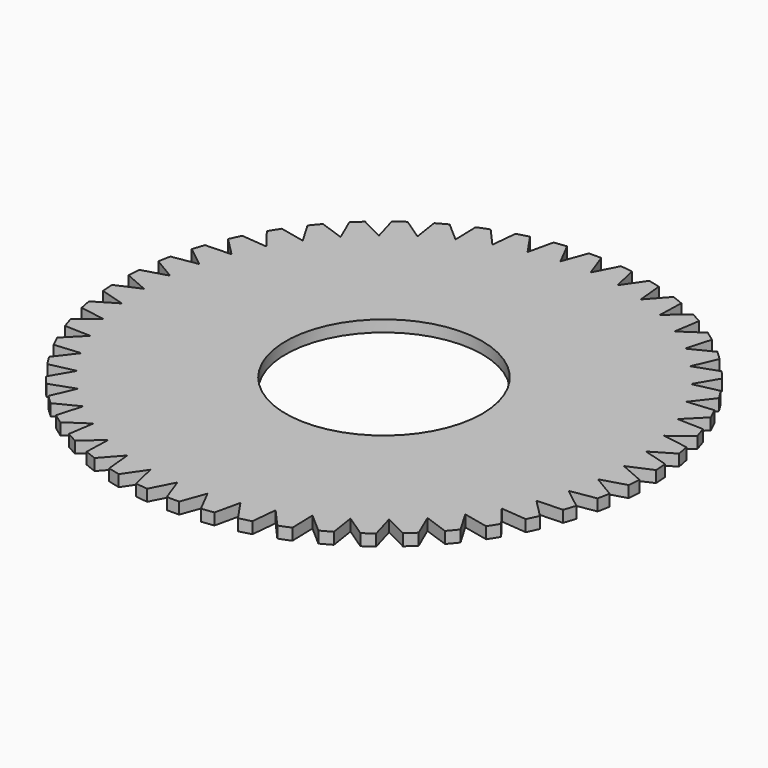
from build123d import *

# Parameters (mm, degrees)
F0_R     = 17.4625
F0_R_2   = 6.5024
F1_DEPTH = 0.762
F3_DEPTH = 0.762


with BuildPart() as f1:
    # F0 (on Top) → F1 (new body)
    with BuildSketch(Plane.XY):
        Circle(F0_R)
        Circle(F0_R_2, mode=Mode.SUBTRACT)
    extrude(amount=F1_DEPTH)

    # F2 (on face) → F3 (cut, through all)
    with BuildSketch(Plane.XY.offset(0.762)):
        with BuildLine():
            Line((17.44898324, 0.6869426038), (15.875, 0))
            Line((15.875, 0), (17.44898324, -0.6869426038))
            ThreePointArc((17.44898324, -0.6869426038), (17.459120483, -0.3435377868), (17.4625, 0))
            ThreePointArc((17.4625, 0), (17.459120483, 0.3435377868), (17.44898324, 0.6869426038))
        make_face()
        with BuildLine():
            Line((17.2252960576, 2.8684633481), (15.7498208834, 1.9896650828))
            Line((15.7498208834, 1.9896650828), (17.3974895332, 1.5054116357))
            ThreePointArc((17.3974895332, 1.5054116357), (17.3645068048, 1.8473791366), (17.3248029717, 2.1886315911))
            ThreePointArc((17.3248029717, 2.1886315911), (17.2783934015, 2.529036914), (17.2252960576, 2.8684633481))
        make_face()
        with BuildLine():
            Line((16.7299556664, 5.0047467118), (15.3762576829, 3.9479519587))
            Line((15.3762576829, 3.9479519587), (17.0716270237, 3.6740246344))
            ThreePointArc((17.0716270237, 3.6740246344), (16.9960444814, 4.0091617875), (16.9138834512, 4.3427471546))
            ThreePointArc((16.9138834512, 4.3427471546), (16.8251757345, 4.6746516184), (16.7299556664, 5.0047467118))
        make_face()
        with BuildLine():
            Line((15.9707738805, 7.0621022302), (14.7602017135, 5.8439772739))
            Line((14.7602017135, 5.8439772739), (16.4765347579, 5.7846960699))
            ThreePointArc((16.4765347579, 5.7846960699), (16.3595443834, 6.1077175619), (16.2362218848, 6.4283750013))
            ThreePointArc((16.2362218848, 6.4283750013), (16.1066149953, 6.7465442742), (15.9707738805, 7.0621022302))
        make_face()
        with BuildLine():
            Line((14.9597234499, 9.0080841777), (13.9113685457, 7.6478395764))
            Line((13.9113685457, 7.6478395764), (15.6215976964, 7.8041393927))
            ThreePointArc((15.6215976964, 7.8041393927), (15.4650444979, 8.1099509819), (15.3025054003, 8.412623534))
            ThreePointArc((15.3025054003, 8.412623534), (15.134043316, 8.7120398966), (14.9597234499, 9.0080841777))
        make_face()
        with BuildLine():
            Line((13.712749244, 10.8120032566), (12.8431447857, 9.3310908801))
            Line((12.8431447857, 9.3310908801), (14.5202987074, 9.7005067753))
            ThreePointArc((14.5202987074, 9.7005067753), (14.3266516222, 9.9842856302), (14.1274592643, 10.2641999682))
            ThreePointArc((14.1274592643, 10.2641999682), (13.9227987329, 10.5401414456), (13.712749244, 10.8120032566))
        make_face()
        with BuildLine():
            Line((12.249516791, 12.4454105853), (11.5723769603, 10.8671853066))
            Line((11.5723769603, 10.8671853066), (13.1900059337, 11.4438913713))
            ThreePointArc((13.1900059337, 11.4438913713), (12.9623188922, 11.7011621298), (12.7296146563, 11.9539038373))
            ThreePointArc((12.7296146563, 11.9539038373), (12.4919832968, 12.2020186676), (12.249516791, 12.4454105853))
        make_face()
        with BuildLine():
            Line((10.5931021406, 13.8825463546), (10.1191058373, 12.2318977291))
            Line((10.1191058373, 12.2318977291), (11.6516988871, 13.0067989641))
            ThreePointArc((11.6516988871, 13.0067989641), (11.3935626498, 13.2335043127), (11.131016421, 13.455087502))
            ThreePointArc((11.131016421, 13.455087502), (10.8641618217, 13.671462766), (10.5931021406, 13.8825463546))
        make_face()
        with BuildLine():
            Line((8.7696279415, 15.1007460749), (8.5062503703, 13.4037058173))
            Line((8.5062503703, 13.4037058173), (9.9296375887, 14.3645815674))
            ThreePointArc((9.9296375887, 14.3645815674), (9.6451231184, 14.5571462273), (9.3568754073, 14.7440763991))
            ThreePointArc((9.3568754073, 14.7440763991), (9.0650060247, 14.9252997297), (8.7696279415, 15.1007460749))
        make_face()
        with BuildLine():
            Line((6.807851471, 16.0807980087), (6.7592462536, 14.3641294579))
            Line((6.7592462536, 14.3641294579), (8.0509799739, 15.4958261384))
            ThreePointArc((8.0509799739, 15.4958261384), (7.7445742336, 15.6512132498), (7.435170879, 15.8005424037))
            ThreePointArc((7.435170879, 15.8005424037), (7.1228896676, 15.9437558007), (6.807851471, 16.0807980087))
        make_face()
        with BuildLine():
            Line((4.7387111161, 16.8072461518), (4.9056447857, 15.0980221962))
            Line((4.9056447857, 15.0980221962), (6.0453535954, 16.3826922744))
            ThreePointArc((6.0453535954, 16.3826922744), (5.7218887868, 16.4984512898), (5.3962092643, 16.6078244158))
            ThreePointArc((5.3962092643, 16.6078244158), (5.0684410854, 16.7107693184), (4.7387111161, 16.8072461518))
        make_face()
        with BuildLine():
            Line((2.594838456, 17.268633983), (2.974678369, 15.5938101053))
            Line((2.974678369, 15.5938101053), (3.9443883794, 17.0111935667))
            ThreePointArc((3.9443883794, 17.0111935667), (3.6089657357, 17.0854988973), (3.272146206, 17.1531911158))
            ThreePointArc((3.272146206, 17.1531911158), (2.9340601595, 17.2142440215), (2.594838456, 17.268633983))
        make_face()
        with BuildLine():
            Line((0.4100436434, 17.4576851404), (0.9967994975, 15.8436743138))
            Line((0.9967994975, 15.8436743138), (1.7812178024, 17.3714181744))
            ThreePointArc((1.7812178024, 17.3714181744), (1.4391271391, 17.4030979808), (1.0964794473, 17.4280417452))
            ThreePointArc((1.0964794473, 17.4280417452), (0.7534073522, 17.446239813), (0.4100436434, 17.4576851404))
        make_face()
        with BuildLine():
            Line((-1.7812178024, 17.3714181744), (-0.9967994975, 15.8436743138))
            Line((-0.9967994975, 15.8436743138), (-0.4100436434, 17.4576851404))
            ThreePointArc((-0.4100436434, 17.4576851404), (-0.7534073522, 17.446239813), (-1.0964794473, 17.4280417452))
            ThreePointArc((-1.0964794473, 17.4280417452), (-1.4391271391, 17.4030979808), (-1.7812178024, 17.3714181744))
        make_face()
        with BuildLine():
            Line((-3.9443883794, 17.0111935667), (-2.974678369, 15.5938101053))
            Line((-2.974678369, 15.5938101053), (-2.594838456, 17.268633983))
            ThreePointArc((-2.594838456, 17.268633983), (-2.9340601595, 17.2142440215), (-3.272146206, 17.1531911158))
            ThreePointArc((-3.272146206, 17.1531911158), (-3.6089657357, 17.0854988973), (-3.9443883794, 17.0111935667))
        make_face()
        with BuildLine():
            Line((-6.0453535954, 16.3826922744), (-4.9056447857, 15.0980221962))
            Line((-4.9056447857, 15.0980221962), (-4.7387111161, 16.8072461518))
            ThreePointArc((-4.7387111161, 16.8072461518), (-5.0684410854, 16.7107693184), (-5.3962092643, 16.6078244158))
            ThreePointArc((-5.3962092643, 16.6078244158), (-5.7218887868, 16.4984512898), (-6.0453535954, 16.3826922744))
        make_face()
        with BuildLine():
            Line((-8.0509799739, 15.4958261384), (-6.7592462536, 14.3641294579))
            Line((-6.7592462536, 14.3641294579), (-6.807851471, 16.0807980087))
            ThreePointArc((-6.807851471, 16.0807980087), (-7.1228896676, 15.9437558007), (-7.435170879, 15.8005424037))
            ThreePointArc((-7.435170879, 15.8005424037), (-7.7445742336, 15.6512132498), (-8.0509799739, 15.4958261384))
        make_face()
        with BuildLine():
            Line((-9.9296375887, 14.3645815674), (-8.5062503703, 13.4037058173))
            Line((-8.5062503703, 13.4037058173), (-8.7696279415, 15.1007460749))
            ThreePointArc((-8.7696279415, 15.1007460749), (-9.0650060247, 14.9252997297), (-9.3568754073, 14.7440763991))
            ThreePointArc((-9.3568754073, 14.7440763991), (-9.6451231184, 14.5571462273), (-9.9296375887, 14.3645815674))
        make_face()
        with BuildLine():
            Line((-11.6516988871, 13.0067989641), (-10.1191058373, 12.2318977291))
            Line((-10.1191058373, 12.2318977291), (-10.5931021406, 13.8825463546))
            ThreePointArc((-10.5931021406, 13.8825463546), (-10.8641618217, 13.671462766), (-11.131016421, 13.455087502))
            ThreePointArc((-11.131016421, 13.455087502), (-11.3935626498, 13.2335043127), (-11.6516988871, 13.0067989641))
        make_face()
        with BuildLine():
            Line((-13.1900059337, 11.4438913713), (-11.5723769603, 10.8671853066))
            Line((-11.5723769603, 10.8671853066), (-12.249516791, 12.4454105853))
            ThreePointArc((-12.249516791, 12.4454105853), (-12.4919832968, 12.2020186676), (-12.7296146563, 11.9539038373))
            ThreePointArc((-12.7296146563, 11.9539038373), (-12.9623188922, 11.7011621298), (-13.1900059337, 11.4438913713))
        make_face()
        with BuildLine():
            Line((-14.5202987074, 9.7005067753), (-12.8431447857, 9.3310908801))
            Line((-12.8431447857, 9.3310908801), (-13.712749244, 10.8120032566))
            ThreePointArc((-13.712749244, 10.8120032566), (-13.9227987329, 10.5401414456), (-14.1274592643, 10.2641999682))
            ThreePointArc((-14.1274592643, 10.2641999682), (-14.3266516222, 9.9842856302), (-14.5202987074, 9.7005067753))
        make_face()
        with BuildLine():
            Line((-15.6215976964, 7.8041393927), (-13.9113685457, 7.6478395764))
            Line((-13.9113685457, 7.6478395764), (-14.9597234499, 9.0080841777))
            ThreePointArc((-14.9597234499, 9.0080841777), (-15.134043316, 8.7120398966), (-15.3025054003, 8.412623534))
            ThreePointArc((-15.3025054003, 8.412623534), (-15.4650444979, 8.1099509819), (-15.6215976964, 7.8041393927))
        make_face()
        with BuildLine():
            Line((-16.4765347579, 5.7846960699), (-14.7602017135, 5.8439772739))
            Line((-14.7602017135, 5.8439772739), (-15.9707738805, 7.0621022302))
            ThreePointArc((-15.9707738805, 7.0621022302), (-16.1066149953, 6.7465442742), (-16.2362218848, 6.4283750013))
            ThreePointArc((-16.2362218848, 6.4283750013), (-16.3595443834, 6.1077175619), (-16.4765347579, 5.7846960699))
        make_face()
        with BuildLine():
            Line((-17.0716270237, 3.6740246344), (-15.3762576829, 3.9479519587))
            Line((-15.3762576829, 3.9479519587), (-16.7299556664, 5.0047467118))
            ThreePointArc((-16.7299556664, 5.0047467118), (-16.8251757345, 4.6746516184), (-16.9138834512, 4.3427471546))
            ThreePointArc((-16.9138834512, 4.3427471546), (-16.9960444814, 4.0091617875), (-17.0716270237, 3.6740246344))
        make_face()
        with BuildLine():
            Line((-17.3974895332, 1.5054116357), (-15.7498208834, 1.9896650828))
            Line((-15.7498208834, 1.9896650828), (-17.2252960576, 2.8684633481))
            ThreePointArc((-17.2252960576, 2.8684633481), (-17.2783934015, 2.529036914), (-17.3248029717, 2.1886315911))
            ThreePointArc((-17.3248029717, 2.1886315911), (-17.3645068048, 1.8473791366), (-17.3974895332, 1.5054116357))
        make_face()
        with BuildLine():
            Line((-17.44898324, -0.6869426038), (-15.875, 0))
            Line((-15.875, 0), (-17.44898324, 0.6869426038))
            ThreePointArc((-17.44898324, 0.6869426038), (-17.459120483, 0.3435377868), (-17.4625, 0))
            ThreePointArc((-17.4625, 0), (-17.459120483, -0.3435377868), (-17.44898324, -0.6869426038))
        make_face()
        with BuildLine():
            Line((-17.2252960576, -2.8684633481), (-15.7498208834, -1.9896650828))
            Line((-15.7498208834, -1.9896650828), (-17.3974895332, -1.5054116357))
            ThreePointArc((-17.3974895332, -1.5054116357), (-17.3645068048, -1.8473791366), (-17.3248029717, -2.1886315911))
            ThreePointArc((-17.3248029717, -2.1886315911), (-17.2783934015, -2.529036914), (-17.2252960576, -2.8684633481))
        make_face()
        with BuildLine():
            Line((-16.7299556664, -5.0047467118), (-15.3762576829, -3.9479519587))
            Line((-15.3762576829, -3.9479519587), (-17.0716270237, -3.6740246344))
            ThreePointArc((-17.0716270237, -3.6740246344), (-16.9960444814, -4.0091617875), (-16.9138834512, -4.3427471546))
            ThreePointArc((-16.9138834512, -4.3427471546), (-16.8251757345, -4.6746516184), (-16.7299556664, -5.0047467118))
        make_face()
        with BuildLine():
            Line((-15.9707738805, -7.0621022302), (-14.7602017135, -5.8439772739))
            Line((-14.7602017135, -5.8439772739), (-16.4765347579, -5.7846960699))
            ThreePointArc((-16.4765347579, -5.7846960699), (-16.3595443834, -6.1077175619), (-16.2362218848, -6.4283750013))
            ThreePointArc((-16.2362218848, -6.4283750013), (-16.1066149953, -6.7465442742), (-15.9707738805, -7.0621022302))
        make_face()
        with BuildLine():
            Line((-14.9597234499, -9.0080841777), (-13.9113685457, -7.6478395764))
            Line((-13.9113685457, -7.6478395764), (-15.6215976964, -7.8041393927))
            ThreePointArc((-15.6215976964, -7.8041393927), (-15.4650444979, -8.1099509819), (-15.3025054003, -8.412623534))
            ThreePointArc((-15.3025054003, -8.412623534), (-15.134043316, -8.7120398966), (-14.9597234499, -9.0080841777))
        make_face()
        with BuildLine():
            Line((-13.712749244, -10.8120032566), (-12.8431447857, -9.3310908801))
            Line((-12.8431447857, -9.3310908801), (-14.5202987074, -9.7005067753))
            ThreePointArc((-14.5202987074, -9.7005067753), (-14.3266516222, -9.9842856302), (-14.1274592643, -10.2641999682))
            ThreePointArc((-14.1274592643, -10.2641999682), (-13.9227987329, -10.5401414456), (-13.712749244, -10.8120032566))
        make_face()
        with BuildLine():
            Line((-12.249516791, -12.4454105853), (-11.5723769603, -10.8671853066))
            Line((-11.5723769603, -10.8671853066), (-13.1900059337, -11.4438913713))
            ThreePointArc((-13.1900059337, -11.4438913713), (-12.9623188922, -11.7011621298), (-12.7296146563, -11.9539038373))
            ThreePointArc((-12.7296146563, -11.9539038373), (-12.4919832968, -12.2020186676), (-12.249516791, -12.4454105853))
        make_face()
        with BuildLine():
            Line((-10.5931021406, -13.8825463546), (-10.1191058373, -12.2318977291))
            Line((-10.1191058373, -12.2318977291), (-11.6516988871, -13.0067989641))
            ThreePointArc((-11.6516988871, -13.0067989641), (-11.3935626498, -13.2335043127), (-11.131016421, -13.455087502))
            ThreePointArc((-11.131016421, -13.455087502), (-10.8641618217, -13.671462766), (-10.5931021406, -13.8825463546))
        make_face()
        with BuildLine():
            Line((-8.7696279415, -15.1007460749), (-8.5062503703, -13.4037058173))
            Line((-8.5062503703, -13.4037058173), (-9.9296375887, -14.3645815674))
            ThreePointArc((-9.9296375887, -14.3645815674), (-9.6451231184, -14.5571462273), (-9.3568754073, -14.7440763991))
            ThreePointArc((-9.3568754073, -14.7440763991), (-9.0650060247, -14.9252997297), (-8.7696279415, -15.1007460749))
        make_face()
        with BuildLine():
            Line((-6.807851471, -16.0807980087), (-6.7592462536, -14.3641294579))
            Line((-6.7592462536, -14.3641294579), (-8.0509799739, -15.4958261384))
            ThreePointArc((-8.0509799739, -15.4958261384), (-7.7445742336, -15.6512132498), (-7.435170879, -15.8005424037))
            ThreePointArc((-7.435170879, -15.8005424037), (-7.1228896676, -15.9437558007), (-6.807851471, -16.0807980087))
        make_face()
        with BuildLine():
            Line((-4.7387111161, -16.8072461518), (-4.9056447857, -15.0980221962))
            Line((-4.9056447857, -15.0980221962), (-6.0453535954, -16.3826922744))
            ThreePointArc((-6.0453535954, -16.3826922744), (-5.7218887868, -16.4984512898), (-5.3962092643, -16.6078244158))
            ThreePointArc((-5.3962092643, -16.6078244158), (-5.0684410854, -16.7107693184), (-4.7387111161, -16.8072461518))
        make_face()
        with BuildLine():
            Line((-2.594838456, -17.268633983), (-2.974678369, -15.5938101053))
            Line((-2.974678369, -15.5938101053), (-3.9443883794, -17.0111935667))
            ThreePointArc((-3.9443883794, -17.0111935667), (-3.6089657357, -17.0854988973), (-3.272146206, -17.1531911158))
            ThreePointArc((-3.272146206, -17.1531911158), (-2.9340601595, -17.2142440215), (-2.594838456, -17.268633983))
        make_face()
        with BuildLine():
            Line((-0.4100436434, -17.4576851404), (-0.9967994975, -15.8436743138))
            Line((-0.9967994975, -15.8436743138), (-1.7812178024, -17.3714181744))
            ThreePointArc((-1.7812178024, -17.3714181744), (-1.4391271391, -17.4030979808), (-1.0964794473, -17.4280417452))
            ThreePointArc((-1.0964794473, -17.4280417452), (-0.7534073522, -17.446239813), (-0.4100436434, -17.4576851404))
        make_face()
        with BuildLine():
            Line((1.7812178024, -17.3714181744), (0.9967994975, -15.8436743138))
            Line((0.9967994975, -15.8436743138), (0.4100436434, -17.4576851404))
            ThreePointArc((0.4100436434, -17.4576851404), (0.7534073522, -17.446239813), (1.0964794473, -17.4280417452))
            ThreePointArc((1.0964794473, -17.4280417452), (1.4391271391, -17.4030979808), (1.7812178024, -17.3714181744))
        make_face()
        with BuildLine():
            Line((3.9443883794, -17.0111935667), (2.974678369, -15.5938101053))
            Line((2.974678369, -15.5938101053), (2.594838456, -17.268633983))
            ThreePointArc((2.594838456, -17.268633983), (2.9340601595, -17.2142440215), (3.272146206, -17.1531911158))
            ThreePointArc((3.272146206, -17.1531911158), (3.6089657357, -17.0854988973), (3.9443883794, -17.0111935667))
        make_face()
        with BuildLine():
            Line((6.0453535954, -16.3826922744), (4.9056447857, -15.0980221962))
            Line((4.9056447857, -15.0980221962), (4.7387111161, -16.8072461518))
            ThreePointArc((4.7387111161, -16.8072461518), (5.0684410854, -16.7107693184), (5.3962092643, -16.6078244158))
            ThreePointArc((5.3962092643, -16.6078244158), (5.7218887868, -16.4984512898), (6.0453535954, -16.3826922744))
        make_face()
        with BuildLine():
            Line((8.0509799739, -15.4958261384), (6.7592462536, -14.3641294579))
            Line((6.7592462536, -14.3641294579), (6.807851471, -16.0807980087))
            ThreePointArc((6.807851471, -16.0807980087), (7.1228896676, -15.9437558007), (7.435170879, -15.8005424037))
            ThreePointArc((7.435170879, -15.8005424037), (7.7445742336, -15.6512132498), (8.0509799739, -15.4958261384))
        make_face()
        with BuildLine():
            Line((9.9296375887, -14.3645815674), (8.5062503703, -13.4037058173))
            Line((8.5062503703, -13.4037058173), (8.7696279415, -15.1007460749))
            ThreePointArc((8.7696279415, -15.1007460749), (9.0650060247, -14.9252997297), (9.3568754073, -14.7440763991))
            ThreePointArc((9.3568754073, -14.7440763991), (9.6451231184, -14.5571462273), (9.9296375887, -14.3645815674))
        make_face()
        with BuildLine():
            Line((11.6516988871, -13.0067989641), (10.1191058373, -12.2318977291))
            Line((10.1191058373, -12.2318977291), (10.5931021406, -13.8825463546))
            ThreePointArc((10.5931021406, -13.8825463546), (10.8641618217, -13.671462766), (11.131016421, -13.455087502))
            ThreePointArc((11.131016421, -13.455087502), (11.3935626498, -13.2335043127), (11.6516988871, -13.0067989641))
        make_face()
        with BuildLine():
            Line((13.1900059337, -11.4438913713), (11.5723769603, -10.8671853066))
            Line((11.5723769603, -10.8671853066), (12.249516791, -12.4454105853))
            ThreePointArc((12.249516791, -12.4454105853), (12.4919832968, -12.2020186676), (12.7296146563, -11.9539038373))
            ThreePointArc((12.7296146563, -11.9539038373), (12.9623188922, -11.7011621298), (13.1900059337, -11.4438913713))
        make_face()
        with BuildLine():
            Line((14.5202987074, -9.7005067753), (12.8431447857, -9.3310908801))
            Line((12.8431447857, -9.3310908801), (13.712749244, -10.8120032566))
            ThreePointArc((13.712749244, -10.8120032566), (13.9227987329, -10.5401414456), (14.1274592643, -10.2641999682))
            ThreePointArc((14.1274592643, -10.2641999682), (14.3266516222, -9.9842856302), (14.5202987074, -9.7005067753))
        make_face()
        with BuildLine():
            Line((15.6215976964, -7.8041393927), (13.9113685457, -7.6478395764))
            Line((13.9113685457, -7.6478395764), (14.9597234499, -9.0080841777))
            ThreePointArc((14.9597234499, -9.0080841777), (15.134043316, -8.7120398966), (15.3025054003, -8.412623534))
            ThreePointArc((15.3025054003, -8.412623534), (15.4650444979, -8.1099509819), (15.6215976964, -7.8041393927))
        make_face()
        with BuildLine():
            Line((16.4765347579, -5.7846960699), (14.7602017135, -5.8439772739))
            Line((14.7602017135, -5.8439772739), (15.9707738805, -7.0621022302))
            ThreePointArc((15.9707738805, -7.0621022302), (16.1066149953, -6.7465442742), (16.2362218848, -6.4283750013))
            ThreePointArc((16.2362218848, -6.4283750013), (16.3595443834, -6.1077175619), (16.4765347579, -5.7846960699))
        make_face()
        with BuildLine():
            Line((17.0716270237, -3.6740246344), (15.3762576829, -3.9479519587))
            Line((15.3762576829, -3.9479519587), (16.7299556664, -5.0047467118))
            ThreePointArc((16.7299556664, -5.0047467118), (16.8251757345, -4.6746516184), (16.9138834512, -4.3427471546))
            ThreePointArc((16.9138834512, -4.3427471546), (16.9960444814, -4.0091617875), (17.0716270237, -3.6740246344))
        make_face()
        with BuildLine():
            Line((17.3974895332, -1.5054116357), (15.7498208834, -1.9896650828))
            Line((15.7498208834, -1.9896650828), (17.2252960576, -2.8684633481))
            ThreePointArc((17.2252960576, -2.8684633481), (17.2783934015, -2.529036914), (17.3248029717, -2.1886315911))
            ThreePointArc((17.3248029717, -2.1886315911), (17.3645068048, -1.8473791366), (17.3974895332, -1.5054116357))
        make_face()
    extrude(amount=-F3_DEPTH, mode=Mode.SUBTRACT)


solid = f1.part
